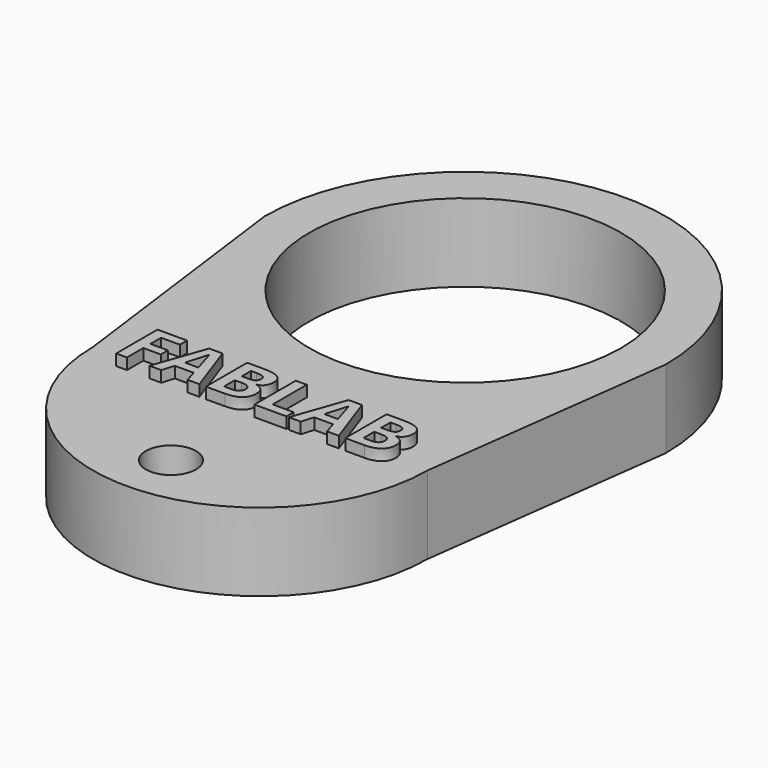
from build123d import *

# Parameters (mm, degrees)
F0_R         = 14
F1_DEPTH     = 7
F2_W         = 19.9
F2_H         = 1.8
F3_DEPTH     = 29
F4_R         = 2.25
F6_DEPTH     = 25
F7_TEXT_SIZE = 6.4937700394
F8_DEPTH     = 1


# Not quite as in the source:
# - Text() gives the source's letters only with a copy of the font that has no kerning and outlines rounded to 1/6400 em; it was checked with that copy


with BuildPart() as f1:
    # F0 (on Top) → F1 (new body)
    with BuildSketch(Plane.XY):
        with BuildLine():
            Line((15, -23), (18, 0))
            ThreePointArc((18, 0), (0, 18), (-18, 0))
            Line((-18, 0), (-15, -23))
            ThreePointArc((-15, -23), (0, -38), (15, -23))
        make_face()
        Circle(F0_R, mode=Mode.SUBTRACT)
    extrude(amount=F1_DEPTH)

    # F2 (on Front) → F3 (cut)
    with BuildSketch(Plane.XZ):
        with Locations((0, 3.5)):
            Rectangle(F2_W, F2_H)
    extrude(amount=F3_DEPTH, mode=Mode.SUBTRACT)

    # F4 (on face) → F6 (cut)
    with BuildSketch(Plane.XY.offset(7)):
        with Locations((0, -33)):
            Circle(F4_R)
    extrude(amount=-F6_DEPTH, mode=Mode.SUBTRACT)

    # F7 (on face) → F8 (join)
    with BuildSketch(Plane.XY.offset(7)):
        with Locations((-12.5, -24.2458250778)):
            Text('FABLAB', F7_TEXT_SIZE, font='Open Sans', font_style=FontStyle.BOLD, text_align=(TextAlign.LEFT, TextAlign.BOTTOM))
    extrude(amount=F8_DEPTH)


solid = f1.part
